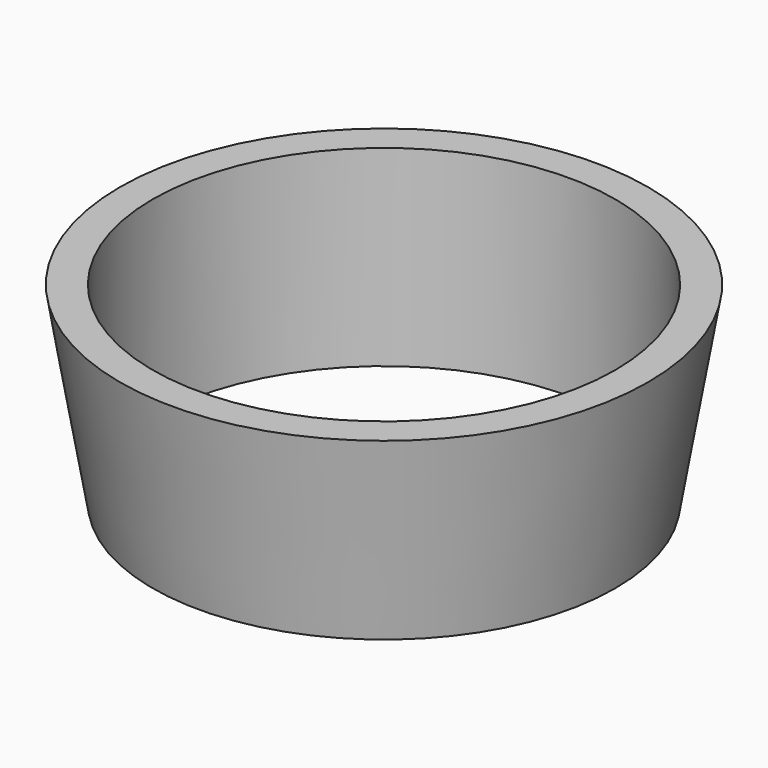
from build123d import *

# Parameters (mm, degrees)
F0_R     = 30.578115114
F1_DEPTH = 25.4
F1_TAPER = -9.7
F3_DEPTH = 25.4


# Not quite as in the source:
# - a feature of the source that left no trace in its solid (it failed there, or was rolled back) is left out


with BuildPart() as f1:
    # F0 (on Top) → F1 (new body)
    with BuildSketch(Plane.XY):
        with Locations((-103.9689183235, 0)):
            Circle(F0_R)
    extrude(amount=F1_DEPTH, taper=F1_TAPER)

    # F0 (on Top) → F3 (cut)
    with BuildSketch(Plane.XY):
        with Locations((-103.9689183235, 0)):
            Circle(F0_R)
    extrude(amount=F3_DEPTH, mode=Mode.SUBTRACT)


solid = f1.part
